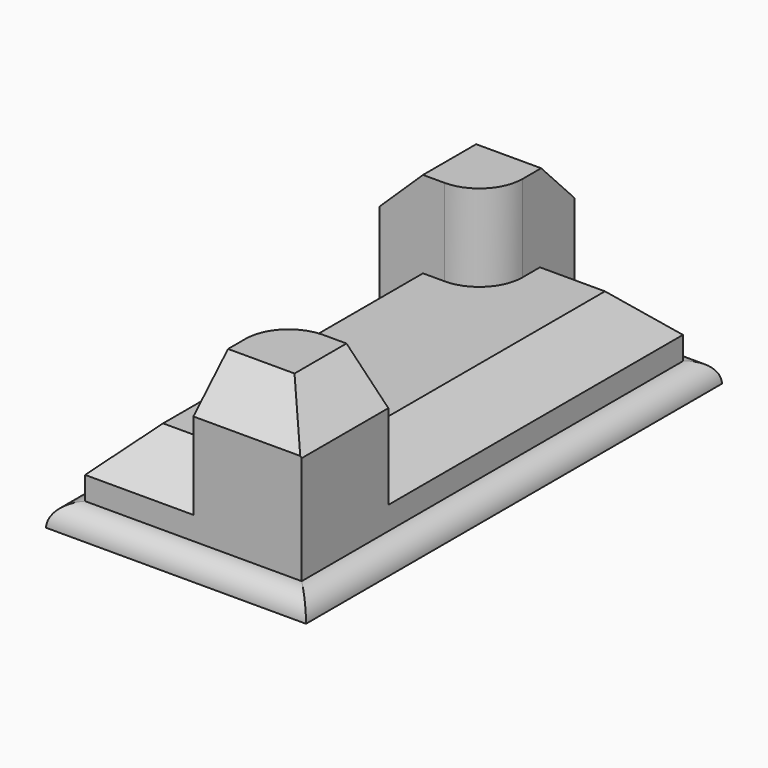
from build123d import *

# Parameters (mm, degrees)
F0_W        = 76.2
F0_H        = 152.4
F1_DEPTH    = 6.35
F2_DEPTH    = 25.4
F3_DEPTH    = 50.8
F4_C1_SIZE2 = 12.7
F4_C1_SIZE  = 12.26424744
F4_C2_SIZE2 = 12.7
F4_C2_SIZE  = 12.26424744
F4_C3_SIZE2 = 12.26424744
F4_C3_SIZE  = 12.7
F4_C4_SIZE2 = 12.7
F4_C4_SIZE  = 12.26424744
F4_C5_SIZE2 = 12.26424744
F4_C5_SIZE  = 12.7
F4_C6_SIZE2 = 12.26424744
F4_C6_SIZE  = 12.7
F4_C7_SIZE2 = 12.26424744
F4_C7_SIZE  = 12.7
F4_C8_SIZE2 = 12.26424744
F4_C8_SIZE  = 12.7
F5_R        = 6.34999


# Not quite as in the source:
# - a fillet or chamfer is up to 0.001 mm smaller than in the source, because OpenCascade refuses the exact size


with BuildPart() as f1:
    # F0 (on Top) → F1 (new body)
    with BuildSketch(Plane.XY):
        with Locations((0, -69.85)):
            Rectangle(F0_W, F0_H)
        Polygon((-31.75, -31.75), (-31.75, 0), (0, 0), (31.75, 0), (31.75, -107.95), (31.75, -139.7), (0, -139.7), (-31.75, -139.7), align=None, mode=Mode.SUBTRACT)
    extrude(amount=F1_DEPTH)

    # F0 (on Top) → F2 (join)
    with BuildSketch(Plane.XY):
        with BuildLine():
            Line((31.75, 0), (0, 0))
            Line((0, 0), (0, -19.05))
            ThreePointArc((0, -19.05), (-3.7197438789, -28.0302561211), (-12.7, -31.75))
            Line((-12.7, -31.75), (-31.75, -31.75))
            Line((-31.75, -31.75), (-31.75, -139.7))
            Line((-31.75, -139.7), (0, -139.7))
            Line((0, -139.7), (0, -120.65))
            ThreePointArc((0, -120.65), (3.7197438789, -111.6697438789), (12.7, -107.95))
            Line((12.7, -107.95), (31.75, -107.95))
            Line((31.75, -107.95), (31.75, 0))
        make_face()
    extrude(amount=F2_DEPTH)

    # F0 (on Top) → F3 (join)
    with BuildSketch(Plane.XY):
        with BuildLine():
            Line((0, 0), (-31.75, 0))
            Line((-31.75, 0), (-31.75, -31.75))
            Line((-31.75, -31.75), (-12.7, -31.75))
            ThreePointArc((-12.7, -31.75), (-3.7197438789, -28.0302561211), (0, -19.05))
            Line((0, -19.05), (0, 0))
        make_face()
        with BuildLine():
            Line((31.75, -139.7), (31.75, -107.95))
            Line((31.75, -107.95), (12.7, -107.95))
            ThreePointArc((12.7, -107.95), (3.7197438789, -111.6697438789), (0, -120.65))
            Line((0, -120.65), (0, -139.7))
            Line((0, -139.7), (31.75, -139.7))
        make_face()
    extrude(amount=F3_DEPTH)

    # F4: chamfer of 12.7 x 12.26424744 on 8 edges, made by hand

    # F4_c1
    f4_c1_edges = [f1.edges().sort_by_distance(p)[0] for p in [
        (-15.875, -139.7, 25.4),
    ]]
    f4_c1_side = f1.faces().sort_by_distance((-15.875, -139.7, 25.1547150512))[0]
    chamfer(f4_c1_edges, length=F4_C1_SIZE, length2=F4_C1_SIZE2, reference=f4_c1_side)

    # F4_c2
    f4_c2_edges = [f1.edges().sort_by_distance(p)[0] for p in [
        (15.875, -139.7, 50.8),
    ]]
    f4_c2_side = f1.faces().sort_by_distance((15.875, -139.7, 50.5547150512))[0]
    chamfer(f4_c2_edges, length=F4_C2_SIZE, length2=F4_C2_SIZE2, reference=f4_c2_side)

    # F4_c3
    f4_c3_edges = [f1.edges().sort_by_distance(p)[0] for p in [
        (31.75, -117.475, 50.8),
    ]]
    f4_c3_side = f1.faces().sort_by_distance((31.75, -117.475, 50.5547150512))[0]
    chamfer(f4_c3_edges, length=F4_C3_SIZE, length2=F4_C3_SIZE2, reference=f4_c3_side)

    # F4_c4
    f4_c4_edges = [f1.edges().sort_by_distance(p)[0] for p in [
        (15.875, 0, 25.4),
    ]]
    f4_c4_side = f1.faces().sort_by_distance((15.875, 0, 25.1547150512))[0]
    chamfer(f4_c4_edges, length=F4_C4_SIZE, length2=F4_C4_SIZE2, reference=f4_c4_side)

    # F4_c5
    f4_c5_edges = [f1.edges().sort_by_distance(p)[0] for p in [
        (-31.75, -79.375, 25.4),
    ]]
    f4_c5_side = f1.faces().sort_by_distance((-31.5047150512, -79.375, 25.4))[0]
    chamfer(f4_c5_edges, length=F4_C5_SIZE, length2=F4_C5_SIZE2, reference=f4_c5_side)

    # F4_c6
    f4_c6_edges = [f1.edges().sort_by_distance(p)[0] for p in [
        (31.75, -60.325, 25.4),
    ]]
    f4_c6_side = f1.faces().sort_by_distance((31.5047150512, -60.325, 25.4))[0]
    chamfer(f4_c6_edges, length=F4_C6_SIZE, length2=F4_C6_SIZE2, reference=f4_c6_side)

    # F4_c7
    f4_c7_edges = [f1.edges().sort_by_distance(p)[0] for p in [
        (-15.875, 0, 50.8),
    ]]
    f4_c7_side = f1.faces().sort_by_distance((-15.875, 0, 50.5547150512))[0]
    chamfer(f4_c7_edges, length=F4_C7_SIZE, length2=F4_C7_SIZE2, reference=f4_c7_side)

    # F4_c8
    f4_c8_edges = [f1.edges().sort_by_distance(p)[0] for p in [
        (-31.75, -22.00712372, 50.8),
    ]]
    f4_c8_side = f1.faces().sort_by_distance((-31.5047150512, -22.00712372, 50.8))[0]
    chamfer(f4_c8_edges, length=F4_C8_SIZE, length2=F4_C8_SIZE2, reference=f4_c8_side)

    # F5 (radius 6.35 in the source; OpenCascade refuses exactly that, so slightly less here)
    f5_edges = [f1.edges().sort_by_distance(p)[0] for p in [
        (38.1, -69.85, 6.35),
        (0, 6.35, 6.35),
        (-38.1, -69.85, 6.35),
        (0, -146.05, 6.35),
    ]]
    fillet(f5_edges, radius=F5_R)


solid = f1.part
